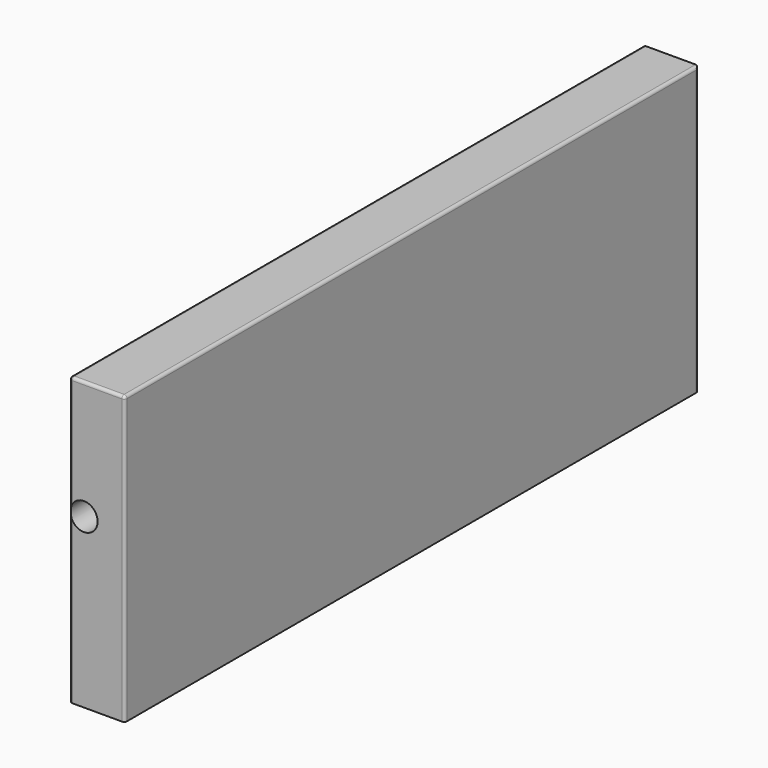
from build123d import *

# Parameters (mm, degrees)
F0_W         = 97.7746620774
F0_H         = 1270
F1_DEPTH     = 508
F2_R         = 24.2123900656
F3_DEPTH     = 762
F4_T1_DEPTH  = 87.6146620774
F4_T3_DEPTH  = 1277.62
F4_T5_DEPTH  = 515.62
F4_T7_DEPTH  = 533.4
F4_S11_W     = 5.08
F4_S11_H     = 5.08
F4_T12_DEPTH = 5.08
F4_S17_W     = 5.08
F4_S17_H     = 5.08
F4_T18_DEPTH = 5.08


# Not quite as in the source:
# - a fillet or chamfer that OpenCascade refuses, or shapes differently, is made with other operations: its cross-section is extruded or revolved along the edge and cut away or added


with BuildPart() as f1:
    # F0 (on Top) → F1 (new body)
    with BuildSketch(Plane.XY):
        with Locations((-1.3020187616, 606.1489956826)):
            Rectangle(F0_W, F0_H)
    extrude(amount=F1_DEPTH)

    # F2 (on face) → F3 (cut)
    with BuildSketch(Plane.XZ.offset(28.8510043174)):
        with Locations((-24.6240980923, 297.7288961411)):
            Circle(F2_R)
    extrude(amount=-F3_DEPTH, mode=Mode.SUBTRACT)

    # F4: fillet of radius 5.08 on 6 edges, made by hand

    # F4_s2 → F4_t1 (cut)
    with BuildSketch(Plane.YZ.offset(-45.1093498003)):
        with BuildLine():
            ThreePointArc((-23.7710043174, 508), (-27.3631067658, 506.5121024484), (-28.8510043174, 502.92))
            Line((-28.8510043174, 502.92), (-28.8510043174, 508))
            Line((-28.8510043174, 508), (-23.7710043174, 508))
        make_face()
    extrude(amount=F4_T1_DEPTH, mode=Mode.SUBTRACT)

    # F4_s4 → F4_t3 (cut)
    with BuildSketch(Plane.XZ.offset(-1253.8489956826)):
        with BuildLine():
            ThreePointArc((47.5853122771, 502.92), (46.0974147255, 506.5121024484), (42.5053122771, 508))
            Line((42.5053122771, 508), (47.5853122771, 508))
            Line((47.5853122771, 508), (47.5853122771, 502.92))
        make_face()
        with BuildLine():
            ThreePointArc((-50.1893498003, 502.92), (-48.7014522488, 506.5121024484), (-45.1093498003, 508))
            Line((-45.1093498003, 508), (-50.1893498003, 508))
            Line((-50.1893498003, 508), (-50.1893498003, 502.92))
        make_face()
    extrude(amount=F4_T3_DEPTH, mode=Mode.SUBTRACT)

    # F4_s6 → F4_t5 (cut)
    with BuildSketch(Plane.XY.offset(-12.7)):
        with BuildLine():
            ThreePointArc((47.5853122771, -23.7710043174), (46.0974147255, -27.3631067658), (42.5053122771, -28.8510043174))
            Line((42.5053122771, -28.8510043174), (47.5853122771, -28.8510043174))
            Line((47.5853122771, -28.8510043174), (47.5853122771, -23.7710043174))
        make_face()
        with BuildLine():
            ThreePointArc((-50.1893498003, -23.7710043174), (-48.7014522488, -27.3631067658), (-45.1093498003, -28.8510043174))
            Line((-45.1093498003, -28.8510043174), (-50.1893498003, -28.8510043174))
            Line((-50.1893498003, -28.8510043174), (-50.1893498003, -23.7710043174))
        make_face()
    extrude(amount=F4_T5_DEPTH, mode=Mode.SUBTRACT)

    # F4_s8 → F4_t7 (cut)
    with BuildSketch(Plane.XY.offset(-12.7)):
        with BuildLine():
            ThreePointArc((42.5053122771, 1241.1489956826), (46.0974147255, 1239.661098131), (47.5853122771, 1236.0689956826))
            Line((47.5853122771, 1236.0689956826), (47.5853122771, 1241.1489956826))
            Line((47.5853122771, 1241.1489956826), (42.5053122771, 1241.1489956826))
        make_face()
    extrude(amount=F4_T7_DEPTH, mode=Mode.SUBTRACT)


with BuildPart() as f4_tool10:
    # F4_s11 → F4_t12 (new body)
    with BuildSketch(Plane.YZ.offset(-45.1093498003)):
        with Locations((-26.3110043174, 505.46)):
            Rectangle(F4_S11_W, F4_S11_H)
    extrude(amount=-F4_T12_DEPTH)

    # F4_s13 → F4_t14 (revolve, cut)
    with BuildSketch(Plane(origin=(-45.1093498003, -23.7710043174, 502.92), x_dir=(0, 0.7071067812, -0.7071067812), z_dir=(0, 0.7071067812, 0.7071067812))):
        with BuildLine():
            ThreePointArc((0, -5.08), (5.08, 0), (0, 5.08))
            Line((0, 5.08), (0, -5.08))
        make_face()
    revolve(axis=Axis((-45.1093498003, -23.7710043174, 502.92), (-1, 0, 0)), mode=Mode.SUBTRACT)


with BuildPart() as f1_1:
    add(f1.part)

    # F4_t9: cut F4_tool10
    add(f4_tool10.part, mode=Mode.SUBTRACT)


with BuildPart() as f4_tool16:
    # F4_s17 → F4_t18 (new body)
    with BuildSketch(Plane.YZ.offset(42.5053122771)):
        with Locations((-26.3110043174, 505.46)):
            Rectangle(F4_S17_W, F4_S17_H)
    extrude(amount=F4_T18_DEPTH)

    # F4_s19 → F4_t20 (revolve, cut)
    with BuildSketch(Plane(origin=(42.5053122771, -23.7710043174, 502.92), x_dir=(0, 0.7071067812, -0.7071067812), z_dir=(0, -0.7071067812, -0.7071067812))):
        with BuildLine():
            ThreePointArc((0, -5.08), (5.08, 0), (0, 5.08))
            Line((0, 5.08), (0, -5.08))
        make_face()
    revolve(axis=Axis((42.5053122771, -23.7710043174, 502.92), (1, 0, 0)), mode=Mode.SUBTRACT)


with BuildPart() as f1_2:
    add(f1_1.part)

    # F4_t15: cut F4_tool16
    add(f4_tool16.part, mode=Mode.SUBTRACT)


solid = f1_2.part
